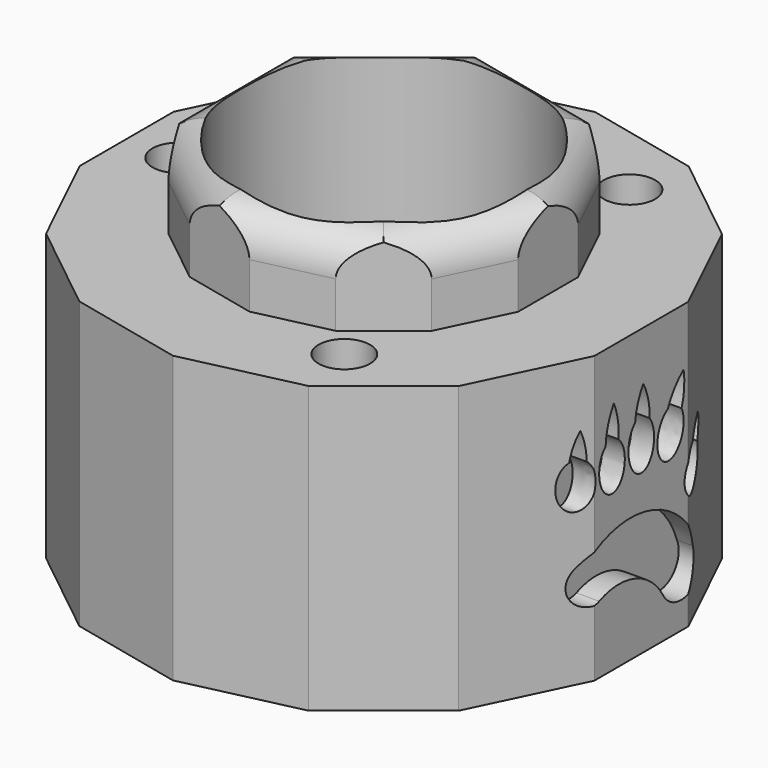
from build123d import *

# Parameters (mm, degrees)
F0_R         = 12.5
F1_DEPTH     = 12.5
F2_R         = 2.25
F3_DEPTH     = 25
F4_R         = 12.5
F5_DEPTH     = 7.5
F6_T1_DEPTH  = 24.050587715
F6_T3_DEPTH  = 24.050587715
F6_T5_DEPTH  = 24.050587715
F6_T7_DEPTH  = 24.050587715
F6_T9_DEPTH  = 24.050587715
F6_T11_DEPTH = 24.050587715
F6_T13_DEPTH = 24.050587715
F8_DEPTH     = 2


# Not quite as in the source:
# - a fillet or chamfer that OpenCascade refuses, or shapes differently, is made with other operations: its cross-section is extruded or revolved along the edge and cut away or added


with BuildPart() as f1:
    # F0 (on Top) → F1 (new body, symmetric)
    with BuildSketch(Plane.XY):
        Polygon((22.5, -5.1354781738), (22.5, 5.1354781738), (18.0435990556, 14.3892900865), (10.013442028, 20.7931266245), (0, 23.0786294236), (-10.013442028, 20.7931266245), (-18.0435990556, 14.3892900865), (-22.5, 5.1354781738), (-22.5, -5.1354781738), (-18.0435990556, -14.3892900865), (-10.013442028, -20.7931266245), (0, -23.0786294236), (10.013442028, -20.7931266245), (18.0435990556, -14.3892900865), align=None)
        Circle(F0_R, mode=Mode.SUBTRACT)
    extrude(amount=F1_DEPTH, both=True)

    # F2 (on face) → F3 (cut)
    with BuildSketch(Plane.XY.offset(12.5)):
        with Locations((9, 15.5884572681)):
            Circle(F2_R)
        with Locations((-18, 0)):
            Circle(F2_R)
        with Locations((9, -15.5884572681)):
            Circle(F2_R)
    extrude(amount=-F3_DEPTH, mode=Mode.SUBTRACT)

    # F4 (on face) → F5 (join)
    with BuildSketch(Plane.XY.offset(12.5)):
        Polygon((14.35, -3.2752938575), (14.35, 3.2752938575), (11.5078065088, 9.1771694552), (6.3863508045, 13.2613940917), (0, 14.719036988), (-6.3863508045, 13.2613940917), (-11.5078065088, 9.1771694552), (-14.35, 3.2752938575), (-14.35, -3.2752938575), (-11.5078065088, -9.1771694552), (-6.3863508045, -13.2613940917), (0, -14.719036988), (6.3863508045, -13.2613940917), (11.5078065088, -9.1771694552), align=None)
        Circle(F4_R, mode=Mode.SUBTRACT)
    extrude(amount=F5_DEPTH)

    # F6: fillet of radius 3.5 on 7 edges, made by hand

    # F6_s2 → F6_t1 (cut)
    with BuildSketch(Plane.XZ.offset(-12.0252938575)):
        with BuildLine():
            ThreePointArc((-10.85, 20), (-13.3248737342, 18.9748737342), (-14.35, 16.5))
            Line((-14.35, 16.5), (-14.35, 20))
            Line((-14.35, 20), (-10.85, 20))
        make_face()
    extrude(amount=F6_T1_DEPTH, mode=Mode.SUBTRACT)

    # F6_s4 → F6_t3 (cut)
    with BuildSketch(Plane(origin=(-9.4017533237, 7.4976480845, 0), x_dir=(0, 0, 1), z_dir=(0.7818314825, -0.6234898019, 0))):
        with BuildLine():
            ThreePointArc((20, 10.85), (18.9748737342, 13.3248737342), (16.5, 14.35))
            Line((16.5, 14.35), (20, 14.35))
            Line((20, 14.35), (20, 10.85))
        make_face()
    extrude(amount=F6_T3_DEPTH, mode=Mode.SUBTRACT)

    # F6_s6 → F6_t5 (cut)
    with BuildSketch(Plane(origin=(-11.7237946339, -2.6758796203, 0), x_dir=(0, 0, 1), z_dir=(0.9749279122, 0.222520934, 0))):
        with BuildLine():
            ThreePointArc((20, 10.85), (18.9748737342, 13.3248737342), (16.5, 14.35))
            Line((16.5, 14.35), (20, 14.35))
            Line((20, 14.35), (20, 10.85))
        make_face()
    extrude(amount=F6_T5_DEPTH, mode=Mode.SUBTRACT)

    # F6_s8 → F6_t7 (cut)
    with BuildSketch(Plane(origin=(-5.2175794629, -10.834415393, 0), x_dir=(0, 0, 1), z_dir=(0.4338837391, 0.9009688679, 0))):
        with BuildLine():
            ThreePointArc((20, 10.85), (18.9748737342, 13.3248737342), (16.5, 14.35))
            Line((16.5, 14.35), (20, 14.35))
            Line((20, 14.35), (20, 10.85))
        make_face()
    extrude(amount=F6_T7_DEPTH, mode=Mode.SUBTRACT)

    # F6_s10 → F6_t9 (cut)
    with BuildSketch(Plane(origin=(5.2175794629, -10.834415393, 0), x_dir=(0, 0, 1), z_dir=(-0.4338837391, 0.9009688679, 0))):
        with BuildLine():
            ThreePointArc((20, 10.85), (18.9748737342, 13.3248737342), (16.5, 14.35))
            Line((16.5, 14.35), (20, 14.35))
            Line((20, 14.35), (20, 10.85))
        make_face()
    extrude(amount=F6_T9_DEPTH, mode=Mode.SUBTRACT)

    # F6_s12 → F6_t11 (cut)
    with BuildSketch(Plane(origin=(11.7237946339, -2.6758796203, 0), x_dir=(0, 0, 1), z_dir=(-0.9749279122, 0.222520934, 0))):
        with BuildLine():
            ThreePointArc((20, 10.85), (18.9748737342, 13.3248737342), (16.5, 14.35))
            Line((16.5, 14.35), (20, 14.35))
            Line((20, 14.35), (20, 10.85))
        make_face()
    extrude(amount=F6_T11_DEPTH, mode=Mode.SUBTRACT)

    # F6_s14 → F6_t13 (cut)
    with BuildSketch(Plane(origin=(9.4017533237, 7.4976480845, 0), x_dir=(0, 0, 1), z_dir=(-0.7818314825, -0.6234898019, 0))):
        with BuildLine():
            ThreePointArc((20, 10.85), (18.9748737342, 13.3248737342), (16.5, 14.35))
            Line((16.5, 14.35), (20, 14.35))
            Line((20, 14.35), (20, 10.85))
        make_face()
    extrude(amount=F6_T13_DEPTH, mode=Mode.SUBTRACT)

    # F7 (on face) → F8 (cut)
    with BuildSketch(Plane.YZ.offset(22.5)):
        with BuildLine():
            ThreePointArc((-6.08032713, 7), (-6.5709395266, 5.8842188275), (-6.8446164746, 4.6964608232))
            add(Edge.make_bspline(
                [(-6.8446164746, 4.6964608232), (-8.5118431653, 3.8987596156), (-7.5942066586, 1.756193723), (-6.676570152, -0.3863721695), (-5.4204160797, 1.3711319286), (-4.1642620074, 3.1286360267), (-5.6446164746, 4.4838947381)],
                knots=[3.4647722977, 3.4647722977, 3.4647722977, 5.2614695117, 5.2614695117, 7.0581667257, 7.0581667257, 8.8548639397, 8.8548639397, 8.8548639397], degree=2, weights=[1, 0.6229027007, 1, 0.6229027007, 1, 0.6229027007, 1]))
            ThreePointArc((-5.6446164746, 4.4838947381), (-5.761433535, 5.7594440336), (-6.08032713, 7))
        make_face()
        with BuildLine():
            ThreePointArc((-3, 8), (-3.6341058947, 6.5649040102), (-3.9, 5.0186533479))
            add(Edge.make_bspline(
                [(-3.9, 5.0186533479), (-5.3449244407, 3.7673120757), (-4.2724622204, 1.8501460197), (-3.2, -0.0670200364), (-2.1275377796, 1.8501460197), (-1.0550755593, 3.7673120757), (-2.5, 5.0186533479)],
                knots=[3.6651914292, 3.6651914292, 3.6651914292, 5.4105206812, 5.4105206812, 7.1558499332, 7.1558499332, 8.9011791852, 8.9011791852, 8.9011791852], degree=2, weights=[1, 0.6427876097, 1, 0.6427876097, 1, 0.6427876097, 1]))
            ThreePointArc((-2.5, 5.0186533479), (-2.5591609645, 6.5413321832), (-3, 8))
        make_face()
        with BuildLine():
            ThreePointArc((0.2275558291, 8.2), (-0.3814401497, 6.9183905981), (-0.6724441709, 5.5296086062))
            add(Edge.make_bspline(
                [(-0.6724441709, 5.5296086062), (-4.5551319088, 2.1883602337), (-0.1559076785, 1.4136843578), (4.2433165517, 0.6390084818), (0.9275558291, 5.247858612)],
                knots=[3.6426090527, 3.6426090527, 3.6426090527, 6.1715912058, 6.1715912058, 8.7005733589, 8.7005733589, 8.7005733589], degree=2, weights=[1, 0.301537928, 1, 0.301537928, 1]))
            ThreePointArc((0.9275558291, 5.247858612), (0.7672369702, 6.7689057422), (0.2275558291, 8.2))
        make_face()
        with BuildLine():
            ThreePointArc((4.6275558291, 7.5), (3.6127003085, 6.4223734822), (2.8925635541, 5.1290778105))
            add(Edge.make_bspline(
                [(2.8925635541, 5.1290778105), (-1.6007345704, 2.6680437483), (2.6559421174, 1.1765704347), (6.9126188052, -0.3149028789), (4.4025558291, 4.6)],
                knots=[3.6564949123, 3.6564949123, 3.6564949123, 6.1933168635, 6.1933168635, 8.7301388146, 8.7301388146, 8.7301388146], degree=2, weights=[1, 0.2977981768, 1, 0.2977981768, 1]))
            ThreePointArc((4.4025558291, 4.6), (4.6934507475, 6.036159015), (4.6275558291, 7.5))
        make_face()
        with BuildLine():
            ThreePointArc((7.8275558291, 2.635071483), (6.9777355341, 1.9893158846), (6.3875558291, 1.1))
            add(Edge.make_bspline(
                [(6.3875558291, 1.1), (0.8266327144, -0.0014683083), (5.3606005397, -2.5921173467), (9.8945683651, -5.182766385), (7.6126455386, 0.4)],
                knots=[3.5803471544, 3.5803471544, 3.5803471544, 6.1960920441, 6.1960920441, 8.8118369337, 8.8118369337, 8.8118369337], degree=2, weights=[1, 0.2599050592, 1, 0.2599050592, 1]))
            ThreePointArc((7.6126455386, 0.4), (7.89881342, 1.5003518589), (7.8275558291, 2.635071483))
        make_face()
        with BuildLine():
            ThreePointArc((2.4, -9), (5.354892815, -9.90978563), (6.4, -7))
            ThreePointArc((6.4, -7), (0.8632403752, -1.8350585765), (-6.5, -3.6))
            ThreePointArc((-6.5, -3.6), (-6.8228285121, -5.9063339911), (-4.6, -6.6009044571))
            ThreePointArc((-4.6, -6.6009044571), (-0.6410576804, -6.4613658189), (2.4, -9))
        make_face()
    extrude(amount=-F8_DEPTH, mode=Mode.SUBTRACT)


solid = f1.part
